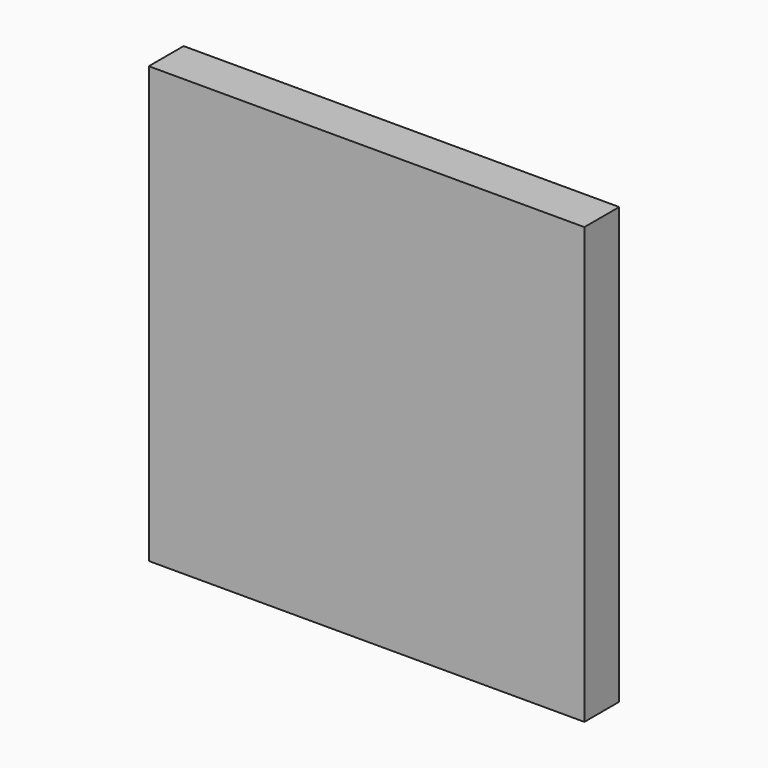
from build123d import *

# Parameters (mm, degrees)
F0_R     = 4.75
F0_R_2   = 1.5
F1_DEPTH = 4
F0_W     = 20
F0_H     = 4
F0_W_2   = 10
F2_DEPTH = 20
F3_R     = 1.6
F4_DEPTH = 4
F5_SIZE  = 3
F6_W     = 160
F6_H     = 160
F6_W_2   = 40
F6_H_2   = 20
F6_R     = 1.6
F7_DEPTH = 16


with BuildPart() as f1:
    # F0 (on Top) → F1 (new body)
    with BuildSketch(Plane.XY):
        Polygon((4, 35), (-4, 35), (-4, 10), (-10, 4), (-10, -21), (-10, -31), (10, -31), (10, -21), (10, 4), (4, 10), align=None)
        with Locations((0, -16)):
            Circle(F0_R, mode=Mode.SUBTRACT)
        with Locations((0, -2)):
            Circle(F0_R, mode=Mode.SUBTRACT)
        with Locations((0, 16)):
            Circle(F0_R_2, mode=Mode.SUBTRACT)
        with Locations((0, 30)):
            Circle(F0_R_2, mode=Mode.SUBTRACT)
        Polygon((-10, -31), (-10, -21), (-20, -31), align=None)
        Polygon((20, -31), (10, -21), (10, -31), align=None)
    extrude(amount=F1_DEPTH)

    # F0 (on Top) → F2 (join)
    with BuildSketch(Plane.XY):
        with Locations((0, -33)):
            Rectangle(F0_W, F0_H)
        with Locations((-15, -33)):
            Rectangle(F0_W_2, F0_H)
        with Locations((15, -33)):
            Rectangle(F0_W_2, F0_H)
    extrude(amount=F2_DEPTH)

    # F3 (on face) → F4 (cut, through all)
    with BuildSketch(Plane(origin=(0, -31, 0), x_dir=(-1, 0, 0), z_dir=(0, 1, 0))):
        with Locations((-15, 12)):
            Circle(F3_R)
        with Locations((15, 12)):
            Circle(F3_R)
    extrude(amount=-F4_DEPTH, mode=Mode.SUBTRACT)

    # F5
    f5_edges = [f1.edges().sort_by_distance(p)[0] for p in [
        (0, -31, 4),
    ]]
    chamfer(f5_edges, length=F5_SIZE)


with BuildPart() as f7:
    # F6 (on face) → F7 (new body)
    with BuildSketch(Plane.XZ.offset(35)):
        Rectangle(F6_W, F6_H)
        with Locations((0, 10)):
            Rectangle(F6_W_2, F6_H_2, mode=Mode.SUBTRACT)
        with Locations((0, 10)):
            Rectangle(F6_W_2, F6_H_2)
        with Locations((-15, 12)):
            Circle(F6_R, mode=Mode.SUBTRACT)
        with Locations((15, 12)):
            Circle(F6_R, mode=Mode.SUBTRACT)
        with Locations((-15, 12)):
            Circle(F6_R)
        with Locations((15, 12)):
            Circle(F6_R)
    extrude(amount=F7_DEPTH)


solid = Compound([f1.part, f7.part])
